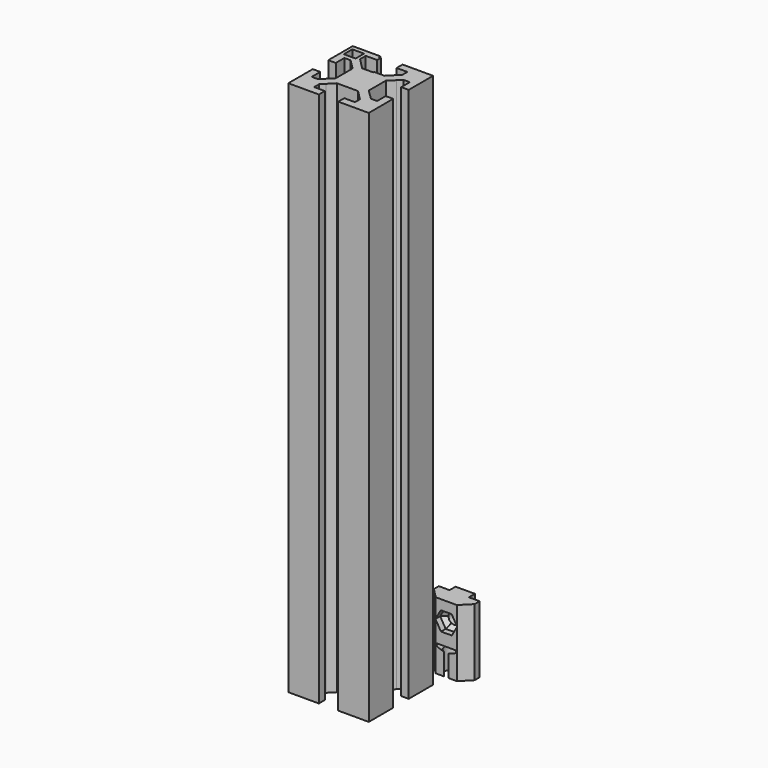
from build123d import *

# Parameters (mm, degrees)
F1_DEPTH     = 25
F2_R         = 2.7
F3_DEPTH     = 10
F4_R         = 2.1
F5_DEPTH     = 3.7
F6_DEPTH     = 25
F7_START     = 8
F2_R_2       = 4.45
F7_DEPTH     = 2
F8_T4_ANGLE  = 359.64
F8_S6_R      = 2.7
F8_T7_DEPTH  = 8
F9_T4_DEPTH  = 11.7565008482
F9_S5_R      = 2.1
F9_T6_DEPTH  = 8
F9_T10_DEPTH = 11.7565008482
F9_S11_R     = 2.1
F9_T12_DEPTH = 8
F9_T16_DEPTH = 11.7565008482
F9_S17_R     = 2.1
F9_T18_DEPTH = 7
F9_T22_DEPTH = 11.7565008482
F9_S23_R     = 2.1
F9_T24_DEPTH = 8
F9_T28_DEPTH = 11.7565008482
F9_S29_R     = 2.1
F9_T30_DEPTH = 7
F9_T34_DEPTH = 11.7565008482
F9_S35_R     = 2.1
F9_T36_DEPTH = 8
F10_W        = 4.3724142015
F10_H        = 3.9559938014
F11_DEPTH    = 200


# Not quite as in the source:
# - a fillet or chamfer that OpenCascade refuses, or shapes differently, is made with other operations: its cross-section is extruded or revolved along the edge and cut away or added


with BuildPart() as f1:
    # F0 (on Top) → F1 (new body)
    with BuildSketch(Plane.XY):
        Polygon((0, 15), (-3.6146675702, 15), (-3.6146675702, 12.2064198286), (-7.6176160946, 12.2064198286), (-7.6176160946, 9.8954397172), (-3.9578238502, 6.1736169547), (0, 6.1736169547), align=None)
        Polygon((3.6146675702, 12.2064198286), (3.6146675702, 15), (0, 15), (0, 6.1736169547), (3.9578238502, 6.1736169547), (7.6176160946, 9.8954397172), (7.6176160946, 12.2064198286), align=None)
    extrude(amount=F1_DEPTH)

    # F2 (on Top) → F3 (cut)
    with BuildSketch(Plane.XY):
        with Locations((0, 8.76147)):
            Circle(F2_R)
    extrude(amount=F3_DEPTH, mode=Mode.SUBTRACT)

    # F4 (on face) → F5 (cut)
    with BuildSketch(Plane.XZ.offset(-6.1736169547)):
        Polygon((2.059832568, 14.396983778), (4.0411979619, 17.9194153968), (1.9813653939, 21.3965439715), (-2.059832568, 21.3512409274), (-4.0411979619, 17.8288093087), (-1.9813653939, 14.3516807339), align=None)
        with Locations((0, 17.8741123527)):
            Circle(F4_R, mode=Mode.SUBTRACT)
    extrude(amount=-F5_DEPTH, mode=Mode.SUBTRACT)

    # F4 (on face) → F6 (cut)
    with BuildSketch(Plane.XZ.offset(-6.1736169547)):
        with Locations((0, 17.8741123527)):
            Circle(F4_R)
    extrude(amount=-F6_DEPTH, mode=Mode.SUBTRACT)

    # F2 (on Top) → F7 (cut)
    with BuildSketch(Plane.XY.offset(F7_START)):
        with Locations((0, 8.76147)):
            Circle(F2_R_2)
        with Locations((0, 8.76147)):
            Circle(F2_R, mode=Mode.SUBTRACT)
        with Locations((0, 8.76147)):
            Circle(F2_R)
    extrude(amount=F7_DEPTH, mode=Mode.SUBTRACT)

    # F8: chamfer of 1.9 x 1.0969655115 on 1 edges, made by hand


with BuildPart() as f8_tool2:
    # F8_s3 → F8_t4 (revolve)
    with BuildSketch(Plane(origin=(0.0275247887, 8.6472e-05, 0), x_dir=(0, 0, 1), z_dir=(-0.9999950652, -0.0031415875, 0))):
        Polygon((9.0969655115, 4.3114267639), (8, 6.2114267639), (8, 4.3114267639), align=None)
    revolve(axis=Axis((0, 8.76147, 8), (0, 0, 1)), revolution_arc=F8_T4_ANGLE)

    split(bisect_by=Plane.XZ.offset(-6.1736169547), keep=Keep.BOTTOM)

    # F8_s6 → F8_t7 (cut, symmetric)
    with BuildSketch(Plane.XY.offset(8.5)):
        with Locations((0, 8.76147)):
            Circle(F8_S6_R)
    extrude(amount=F8_T7_DEPTH, both=True, mode=Mode.SUBTRACT)


with BuildPart() as f1_1:
    add(f1.part)

    # F8_t1: union F8_tool2
    add(f8_tool2.part)

    # F9: chamfer of 1.5 on 6 edges, made by hand


with BuildPart() as f9_tool2:
    # F9_s3 → F9_t4 (new body)
    with BuildSketch(Plane(origin=(-4.8419417128, 0, 8.173506016), x_dir=(0, 1, 0), z_dir=(-0.5096763804, 0, 0.8603661937))):
        Polygon((8.3736169547, -12.610012887), (9.8736169547, -11.110012887), (9.8736169547, -12.610012887), align=None)
    extrude(amount=F9_T4_DEPTH)

    # F9_s5 → F9_t6 (cut, symmetric)
    with BuildSketch(Plane.XZ.offset(-9.1)):
        with Locations((0, 17.8741123527)):
            Circle(F9_S5_R)
    extrude(amount=F9_T6_DEPTH, both=True, mode=Mode.SUBTRACT)


with BuildPart() as f1_2:
    add(f1_1.part)

    # F9_t1: union F9_tool2
    add(f9_tool2.part)


with BuildPart() as f9_tool8:
    # F9_s9 → F9_t10 (new body)
    with BuildSketch(Plane(origin=(4.7557224198, 0, 8.4546278405), x_dir=(0, 1, 0), z_dir=(0.4902607901, 0, 0.87157579))):
        Polygon((9.8736169547, 6.7629764442), (8.3736169547, 5.2629764442), (9.8736169547, 5.2629764442), align=None)
    extrude(amount=F9_T10_DEPTH)

    # F9_s11 → F9_t12 (cut, symmetric)
    with BuildSketch(Plane.XZ.offset(-9.1)):
        with Locations((0, 17.8741123527)):
            Circle(F9_S11_R)
    extrude(amount=F9_T12_DEPTH, both=True, mode=Mode.SUBTRACT)


with BuildPart() as f1_3:
    add(f1_2.part)

    # F9_t7: union F9_tool8
    add(f9_tool8.part)


with BuildPart() as f9_tool14:
    # F9_s15 → F9_t16 (new body)
    with BuildSketch(Plane(origin=(-5.6775321016, 0, -0.0636468417), x_dir=(0, 1, 0), z_dir=(0.9999371705, 0, 0.0112095963))):
        Polygon((9.8736169547, 15.8729893312), (8.3736169547, 14.3729893312), (9.8736169547, 14.3729893312), align=None)
    extrude(amount=F9_T16_DEPTH)

    # F9_s17 → F9_t18 (cut, symmetric)
    with BuildSketch(Plane.XZ.offset(-9.1)):
        with Locations((0, 17.8741123527)):
            Circle(F9_S17_R)
    extrude(amount=F9_T18_DEPTH, both=True, mode=Mode.SUBTRACT)


with BuildPart() as f1_4:
    add(f1_3.part)

    # F9_t13: union F9_tool14
    add(f9_tool14.part)


with BuildPart() as f9_tool20:
    # F9_s21 → F9_t22 (new body)
    with BuildSketch(Plane(origin=(-10.8339525114, 0, 18.288401902), x_dir=(0, 1, 0), z_dir=(0.5096763804, 0, -0.8603661937))):
        Polygon((9.8736169547, 7.110012887), (8.3736169547, 5.610012887), (9.8736169547, 5.610012887), align=None)
    extrude(amount=F9_T22_DEPTH)

    # F9_s23 → F9_t24 (cut, symmetric)
    with BuildSketch(Plane.XZ.offset(-9.1)):
        with Locations((0, 17.8741123527)):
            Circle(F9_S23_R)
    extrude(amount=F9_T24_DEPTH, both=True, mode=Mode.SUBTRACT)


with BuildPart() as f1_5:
    add(f1_4.part)

    # F9_t19: union F9_tool20
    add(f9_tool20.part)


with BuildPart() as f9_tool26:
    # F9_s27 → F9_t28 (new body)
    with BuildSketch(Plane(origin=(6.0782300916, 0, 0.0681387867), x_dir=(0, 1, 0), z_dir=(-0.9999371705, 0, -0.0112095963))):
        Polygon((9.8736169547, -19.8729893312), (8.3736169547, -21.3729893312), (9.8736169547, -21.3729893312), align=None)
    extrude(amount=F9_T28_DEPTH)

    # F9_s29 → F9_t30 (cut, symmetric)
    with BuildSketch(Plane.XZ.offset(-9.1)):
        with Locations((0, 17.8741123527)):
            Circle(F9_S29_R)
    extrude(amount=F9_T30_DEPTH, both=True, mode=Mode.SUBTRACT)


with BuildPart() as f1_6:
    add(f1_5.part)

    # F9_t25: union F9_tool26
    add(f9_tool26.part)


with BuildPart() as f9_tool32:
    # F9_s33 → F9_t34 (new body)
    with BuildSketch(Plane(origin=(10.5194738143, 0, 18.7013093548), x_dir=(0, 1, 0), z_dir=(-0.4902607901, 0, -0.87157579))):
        Polygon((9.8736169547, -10.7629764442), (8.3736169547, -12.2629764442), (9.8736169547, -12.2629764442), align=None)
    extrude(amount=F9_T34_DEPTH)

    # F9_s35 → F9_t36 (cut, symmetric)
    with BuildSketch(Plane.XZ.offset(-9.1)):
        with Locations((0, 17.8741123527)):
            Circle(F9_S35_R)
    extrude(amount=F9_T36_DEPTH, both=True, mode=Mode.SUBTRACT)


with BuildPart() as f1_7:
    add(f1_6.part)

    # F9_t31: union F9_tool32
    add(f9_tool32.part)


with BuildPart() as f11:
    # F10 (on Top) → F11 (new body)
    with BuildSketch(Plane.XY):
        Polygon((-24.939087107, -7.310864791), (-23.4706133497, -8.754863931), (-19.5336121346, -8.754863931), (-23.2350792623, -4.9906599296), (-23.2350792623, -2.3533313495), (-19.00147124, -2.3533313495), (-19.00147124, -0.6182457281), (-19.6261023059, -0.6182457281), (-19.6261023059, 0.0715191143), (-30.0436473898, 0.0715191143), (-30.0436473898, -8.754863931), (-27.2500672184, -8.754863931), (-27.2500672184, -7.310864791), align=None)
        with Locations((-26.6705475635, -3.5678905395)):
            Rectangle(F10_W, F10_H, mode=Mode.SUBTRACT)
        Polygon((-11.0858235396, -21.1020978404), (-6.6166814299, -21.1020978404), (-8.8700304351, -18.8863047359), (-8.8700304351, -10.9706570355), (-8.8700304351, -8.754863931), (-11.0858235396, -8.754863931), (-15.0436473898, -8.754863931), (-15.0436473898, -9.154863931), (-19.1402788162, -9.154863931), (-19.5336121346, -8.754863931), (-23.4706133497, -8.754863931), (-21.2172643445, -10.9706570355), (-21.2172643445, -18.8863047359), (-21.2172643445, -23.3554468456), (-19.00147124, -21.1020978404), align=None)
        Polygon((-27.2500672184, -11.3138133155), (-27.2500672184, -8.754863931), (-30.0436473898, -8.754863931), (-30.0436473898, -10.3460259696), (-30.0436473898, -11.3138133155), align=None)
        Polygon((-8.8700304351, -8.754863931), (-6.6166814299, -8.754863931), (-5.1482076726, -7.310864791), (-2.8372275612, -7.310864791), (-2.8372275612, -8.754863931), (-0.0436473898, -8.754863931), (-0.0436473898, 0.0715191143), (-8.8700304351, 0.0715191143), (-8.8700304351, -2.7220610571), (-7.4260312951, -2.7220610571), (-7.4260312951, -5.0330411685), (-8.8700304351, -6.5015149258), align=None)
        Polygon((-2.8372275612, -11.3138133155), (-0.0436473898, -11.3138133155), (-0.0436473898, -10.3460259696), (-0.0436473898, -8.754863931), (-2.8372275612, -8.754863931), align=None)
        Polygon((-2.8372275612, -21.1020978404), (-0.0436473898, -21.1020978404), (-0.0436473898, -19.5109358018), (-0.0436473898, -18.5431484559), (-2.8372275612, -18.5431484559), align=None)
        Polygon((-10.4611924737, -29.9284808857), (-0.0436473898, -29.9284808857), (-0.0436473898, -21.1020978404), (-2.8372275612, -21.1020978404), (-2.8372275612, -22.5460969803), (-5.1482076726, -22.5460969803), (-6.6166814299, -21.1020978404), (-11.0858235396, -21.1020978404), (-7.4260312951, -24.8239206029), (-7.4260312951, -27.1349007143), (-11.4289798196, -27.1349007143), (-11.4289798196, -29.9284808857), align=None)
        Polygon((-30.0436473898, -29.9284808857), (-21.2172643445, -29.9284808857), (-21.2172643445, -27.1349007143), (-22.6612634844, -27.1349007143), (-22.6612634844, -24.8239206029), (-21.2172643445, -23.3554468456), (-21.2172643445, -18.8863047359), (-24.939087107, -22.5460969803), (-27.2500672184, -22.5460969803), (-27.2500672184, -18.5431484559), (-30.0436473898, -18.5431484559), (-30.0436473898, -19.5109358018), align=None)
        Polygon((-19.6261023059, -29.9284808857), (-18.65831496, -29.9284808857), (-18.65831496, -27.1349007143), (-21.2172643445, -27.1349007143), (-21.2172643445, -29.9284808857), align=None)
        Polygon((-11.4289798196, -2.7220610571), (-8.8700304351, -2.7220610571), (-8.8700304351, 0.0715191143), (-10.4611924737, 0.0715191143), (-11.4289798196, 0.0715191143), align=None)
        Polygon((-11.0858235396, -8.754863931), (-8.8700304351, -8.754863931), (-8.8700304351, -6.5015149258), align=None)
        Polygon((-8.8700304351, -8.754863931), (-8.8700304351, -10.9706570355), (-6.6166814299, -8.754863931), align=None)
    extrude(amount=F11_DEPTH)


solid = Compound([f1_7.part, f11.part])
